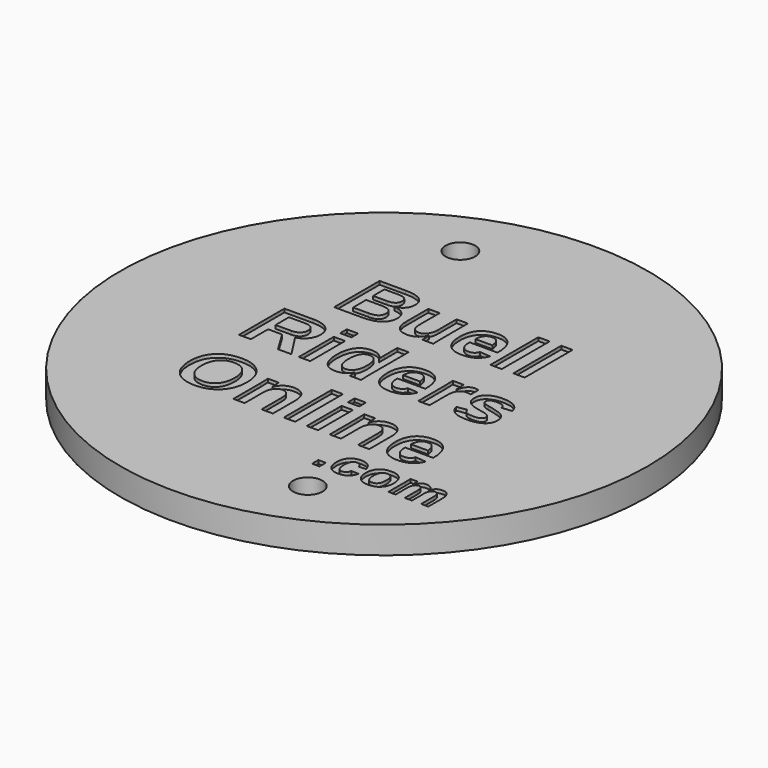
from build123d import *

# Parameters (mm, degrees)
F0_R           = 39.6875
F0_R_2         = 2.2225
F1_DEPTH       = 4.064
F2_TEXT_SIZE   = 12.4192043472
F2_TEXT_SIZE_2 = 7.925912117
F3_DEPTH       = 0.508


# Not quite as in the source:
# - Text() gives the source's letters only with a copy of the font that has no kerning and outlines rounded to 1/6400 em; it was checked with that copy


with BuildPart() as f1:
    # F0 (on Top) → F1 (new body)
    with BuildSketch(Plane.XY):
        Circle(F0_R)
        with Locations((11.674993854, -28.930635052)):
            Circle(F0_R_2, mode=Mode.SUBTRACT)
        with Locations((-11.674993854, 28.930635052)):
            Circle(F0_R_2, mode=Mode.SUBTRACT)
    extrude(amount=F1_DEPTH)

    # F2 (on face) → F3 (cut)
    with BuildSketch(Plane.XY.offset(4.064)):
        with Locations((-15.1718045607, 8.5406689905)):
            Text('Buell', F2_TEXT_SIZE, font='Arimo', font_style=FontStyle.BOLD, text_align=(TextAlign.LEFT, TextAlign.BOTTOM))
        with Locations((-19.5020318265, -3.9343505632)):
            Text('Riders', F2_TEXT_SIZE, font='Arimo', font_style=FontStyle.BOLD, text_align=(TextAlign.LEFT, TextAlign.BOTTOM))
        with Locations((-19.5379310891, -17.0729355887)):
            Text('Online', F2_TEXT_SIZE, font='Arimo', font_style=FontStyle.BOLD, text_align=(TextAlign.LEFT, TextAlign.BOTTOM))
        with Locations((7.9627772793, -24.1537615657)):
            Text('.com', F2_TEXT_SIZE_2, font='Arimo', font_style=FontStyle.BOLD, text_align=(TextAlign.LEFT, TextAlign.BOTTOM))
    extrude(amount=-F3_DEPTH, mode=Mode.SUBTRACT)


solid = f1.part
